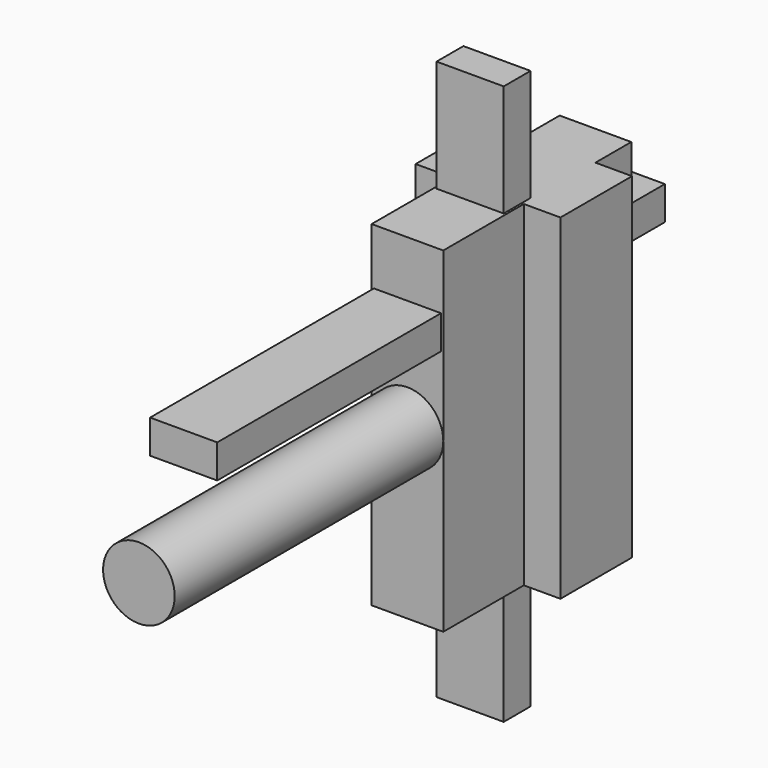
from build123d import *

# Parameters (mm, degrees)
F1_DEPTH = 7.5
F2_R     = 1.6
F3_DEPTH = 15
F4_W     = 3
F4_H     = 1.5
F5_DEPTH = 12.5
F6_W     = 3
F6_H     = 1.5
F7_DEPTH = 12.5


with BuildPart() as f1:
    # F0 (on Top) → F1 (new body, symmetric)
    with BuildSketch(Plane.XY):
        Polygon((1.6, 10.5), (0, 10.5), (-1.6, 10.5), (-1.6, 8.5), (-3.2350461341, 8.5), (-3.2350461341, 4.5), (-1.6, 4.5), (-1.6, 0), (0, 0), (1.6, 0), (1.6, 4.5), (3.2350461341, 4.5), (3.2350461341, 8.5), (1.6, 8.5), align=None)
    extrude(amount=F1_DEPTH, both=True)

    # F2 (on Front) → F3 (join)
    with BuildSketch(Plane.XZ):
        Circle(F2_R)
    extrude(amount=F3_DEPTH)


with BuildPart() as f5:
    # F4 (on Front) → F5 (new body, symmetric)
    with BuildSketch(Plane.XZ):
        with Locations((0, 4.25)):
            Rectangle(F4_W, F4_H)
    extrude(amount=F5_DEPTH, both=True)

    # F6 (on Top) → F7 (join, symmetric)
    with BuildSketch(Plane.XY):
        with Locations((0, 4.25)):
            Rectangle(F6_W, F6_H)
    extrude(amount=F7_DEPTH, both=True)


solid = Compound([f1.part, f5.part])
